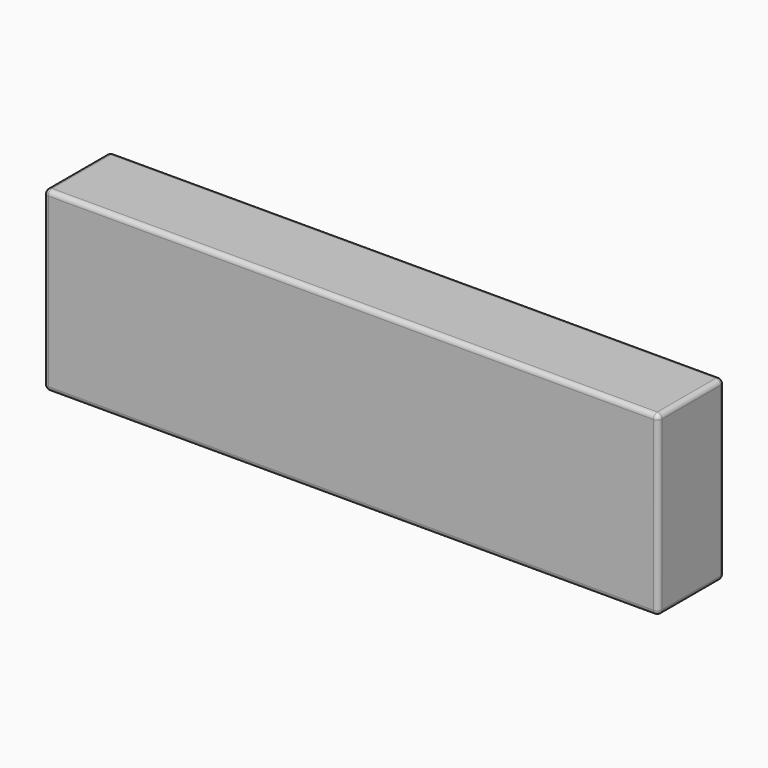
from build123d import *

# Parameters (mm, degrees)
F0_W     = 88.9
F0_H     = 190.5
F1_DEPTH = 330.2
F3_D     = 6.35
F3_DEPTH = 95.251
F4_R     = 5.08


with BuildPart() as f1:
    # F0 (on Right) → F1 (new body, symmetric)
    with BuildSketch(Plane.YZ):
        Rectangle(F0_W, F0_H)
    extrude(amount=F1_DEPTH, both=True)

    # F3 (through all, one way)
    with BuildSketch(Plane.XY):
        with Locations((0, 0)):
            Circle(F3_D / 2)
    extrude(amount=-F3_DEPTH, mode=Mode.SUBTRACT)

    # F4
    f4_edges = [f1.edges().sort_by_distance(p)[0] for p in [
        (0, -44.45, 95.25),
        (0, 44.45, 95.25),
        (330.2, 0, 95.25),
        (330.2, 44.45, 0),
        (330.2, -44.45, 0),
        (330.2, 0, -95.25),
        (0, -44.45, -95.25),
        (0, 44.45, -95.25),
        (-330.2, -44.45, 0),
        (-330.2, 44.45, 0),
        (-330.2, 0, 95.25),
        (-330.2, 0, -95.25),
    ]]
    fillet(f4_edges, radius=F4_R)


solid = f1.part
